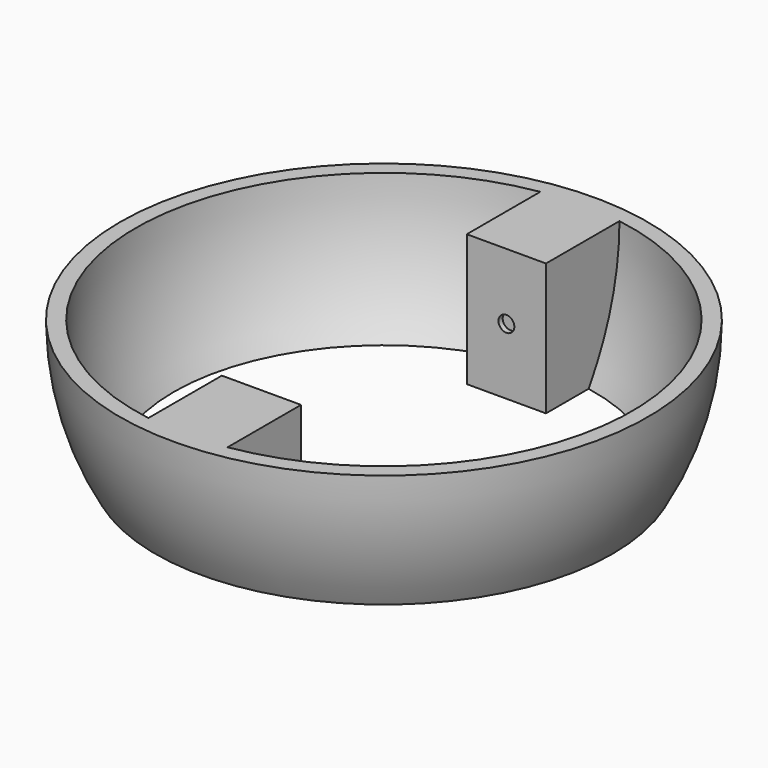
from build123d import *

# Parameters (mm, degrees)
F2_T     = -6
F4_W     = 30
F4_H     = 50
F6_R     = 3
F7_DEPTH = 2


# Not quite as in the source:
# - a pattern or mirror of a feature is missing from the dataset's text; its kind, count and spacing are read off the source's solid


with BuildPart() as f1:
    # F0 (on Front) → F1 (revolve)
    with BuildSketch(Plane.XZ):
        with BuildLine():
            Line((0, 0), (-100, 0))
            ThreePointArc((-100, 0), (-96.5925826289, -25.8819045103), (-86.6025403784, -50))
            Line((-86.6025403784, -50), (0, -50))
            Line((0, -50), (0, 0))
        make_face()
    revolve(axis=Axis((0, 0, -25), (0, 0, -1)))

    # F2
    f2_openings = [f1.faces().sort_by_distance(p)[0] for p in [
        (0, 0, 0),
        (0, 0, -50),
    ]]
    offset(amount=F2_T, openings=f2_openings)

    # F4 (on offset) → F5 (join, up to the next surface of F1)
    with BuildSketch(Plane.XZ.offset(-58)):
        with Locations((0, -25)):
            Rectangle(F4_W, F4_H)
    f5 = extrude(until=Until.NEXT, dir=(0, 1, 0))

    # F5_copies: F5 across plane
    add(f5.mirror(Plane(origin=(0, 0, 0), x_dir=(0, 0, -1), z_dir=(0, -1, 0))))

    # F6 (on face) → F7 (cut)
    with BuildSketch(Plane.XZ.offset(-58)):
        with Locations((0, -25)):
            Circle(F6_R)
    f7 = extrude(amount=-F7_DEPTH, mode=Mode.SUBTRACT)

    # F7_copies: F7 across plane
    add(f7.mirror(Plane(origin=(0, 0, 0), x_dir=(0, 0, -1), z_dir=(0, -1, 0))), mode=Mode.SUBTRACT)


solid = f1.part
